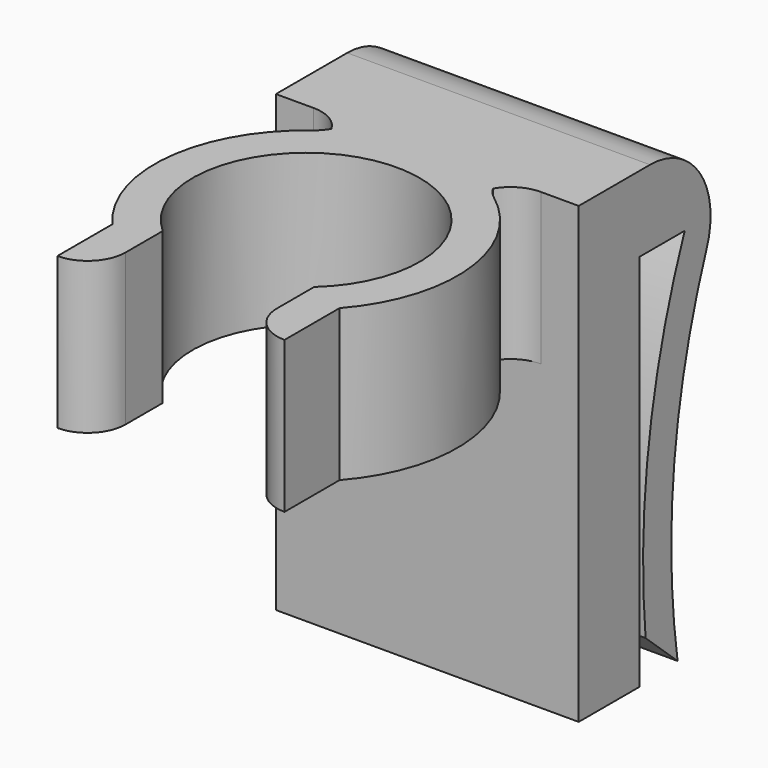
from build123d import *

# Parameters (mm, degrees)
F0_W        = 6.35
F0_H        = 6.35
F0_H_2      = 31.75
F1_DEPTH    = 25.4
F3_DEPTH    = 12.7
F4_R        = 3.17499
F5_T1_DEPTH = 12.7
F6_R        = 6.35
F7_T1_DEPTH = 42.7131376889


# Not quite as in the source:
# - a fillet or chamfer that OpenCascade refuses, or shapes differently, is made with other operations: its cross-section is extruded or revolved along the edge and cut away or added
# - a fillet or chamfer is up to 0.001 mm smaller than in the source, because OpenCascade refuses the exact size


with BuildPart() as f1:
    # F0 (on Right) → F1 (new body)
    with BuildSketch(Plane.YZ):
        with Locations((3.175, 3.175)):
            Rectangle(F0_W, F0_H)
        with Locations((3.175, -15.875)):
            Rectangle(F0_W, F0_H_2)
        with BuildLine():
            Line((6.35, 6.35), (6.35, 0))
            Line((6.35, 0), (11.1125, 0))
            ThreePointArc((11.1125, 0), (7.1582593776, -15.6298064568), (7.4156091525, -31.75))
            Line((7.4156091525, -31.75), (10.4078971116, -31.75))
            ThreePointArc((10.4078971116, -31.75), (10.6800087855, -12.0972684736), (17.4625, 6.35))
            Line((17.4625, 6.35), (6.35, 6.35))
        make_face()
    extrude(amount=F1_DEPTH)

    # F2 (on face) → F3 (join)
    with BuildSketch(Plane.XY.offset(6.35)):
        with BuildLine():
            Line((19.05, 0), (6.35, 0))
            Line((6.35, 0), (6.35, -1.7014773719))
            ThreePointArc((6.35, -1.7014773719), (0.166760111, -10.6486838652), (3.175, -21.1002604126))
            ThreePointArc((3.175, -21.1002604126), (4.6568881715, -22.5284460682), (6.35, -23.6985226281))
            Line((6.35, -23.6985226281), (6.35, -19.7995158286))
            ThreePointArc((6.35, -19.7995158286), (12.7, -3.175), (19.05, -19.7995158286))
            Line((19.05, -19.7995158286), (19.05, -23.6985226281))
            ThreePointArc((19.05, -23.6985226281), (20.7431118285, -22.5284460682), (22.225, -21.1002604126))
            ThreePointArc((22.225, -21.1002604126), (25.233239889, -10.6486838652), (19.05, -1.7014773719))
            Line((19.05, -1.7014773719), (19.05, 0))
        make_face()
        with BuildLine():
            ThreePointArc((6.35, -23.6985226281), (4.6568881715, -22.5284460682), (3.175, -21.1002604126))
            Line((3.175, -21.1002604126), (3.175, -26.8735226281))
            Line((3.175, -26.8735226281), (6.35, -26.8735226281))
            Line((6.35, -26.8735226281), (6.35, -23.6985226281))
        make_face()
        with BuildLine():
            Line((22.225, -26.8735226281), (22.225, -21.1002604126))
            ThreePointArc((22.225, -21.1002604126), (20.7431118285, -22.5284460682), (19.05, -23.6985226281))
            Line((19.05, -23.6985226281), (19.05, -26.8735226281))
            Line((19.05, -26.8735226281), (22.225, -26.8735226281))
        make_face()
    extrude(amount=-F3_DEPTH)

    # F4 (radius 3.175 in the source; OpenCascade refuses exactly that, so slightly less here)
    f4_edges = [f1.edges().sort_by_distance(p)[0] for p in [
        (6.35, -26.873523, 0),
        (19.05, -26.873523, 0),
    ]]
    fillet(f4_edges, radius=F4_R)

    # F5: fillet of radius 3.175 on 4 edges, made by hand

    # F5_s2 → F5_t1 (join)
    with BuildSketch(Plane.XY.offset(-6.35)):
        with BuildLine():
            ThreePointArc((5.08, -2.54), (6.0148063314, -1.4199031657), (6.35, 0))
            Line((6.35, 0), (6.35, -1.7014773719))
            ThreePointArc((6.35, -1.7014773719), (5.7024286321, -2.1016984875), (5.08, -2.54))
        make_face()
        with BuildLine():
            ThreePointArc((20.32, -2.54), (19.3851936686, -1.4199031657), (19.05, 0))
            Line((19.05, 0), (19.05, -1.7014773719))
            ThreePointArc((19.05, -1.7014773719), (19.6975713679, -2.1016984875), (20.32, -2.54))
        make_face()
        with BuildLine():
            ThreePointArc((19.05, -3.175), (19.9799359697, -0.9299359697), (22.225, 0))
            Line((22.225, 0), (19.05, 0))
            Line((19.05, 0), (19.05, -3.175))
        make_face()
        with BuildLine():
            ThreePointArc((3.175, 0), (5.4200640303, -0.9299359697), (6.35, -3.175))
            Line((6.35, -3.175), (6.35, 0))
            Line((6.35, 0), (3.175, 0))
        make_face()
    extrude(amount=F5_T1_DEPTH)

    # F6
    f6_edges = [f1.edges().sort_by_distance(p)[0] for p in [
        (12.7, 17.4625, 6.35),
    ]]
    fillet(f6_edges, radius=F6_R)

    # F7: chamfer of 3.175 on 1 edges, made by hand

    # F7_s2 → F7_t1 (cut)
    with BuildSketch(Plane.YZ.offset(-8.6565688444)):
        with BuildLine():
            Line((10.772273237, -31.8355341736), (6.9175477916, -28.3233800406))
            Line((6.9175477916, -28.3233800406), (6.8543218231, -28.3292729944))
            ThreePointArc((6.8543218231, -28.3292729944), (7.1217830499, -30.0420734544), (7.3528018544, -31.759353786))
            Line((7.3528018544, -31.759353786), (7.4156091525, -31.8135))
            ThreePointArc((7.4156091525, -31.8135), (9.0939411948, -31.8135), (10.772273237, -31.8990341736))
            Line((10.772273237, -31.8990341736), (10.772273237, -31.8355341736))
        make_face()
    extrude(amount=F7_T1_DEPTH, mode=Mode.SUBTRACT)


solid = f1.part
